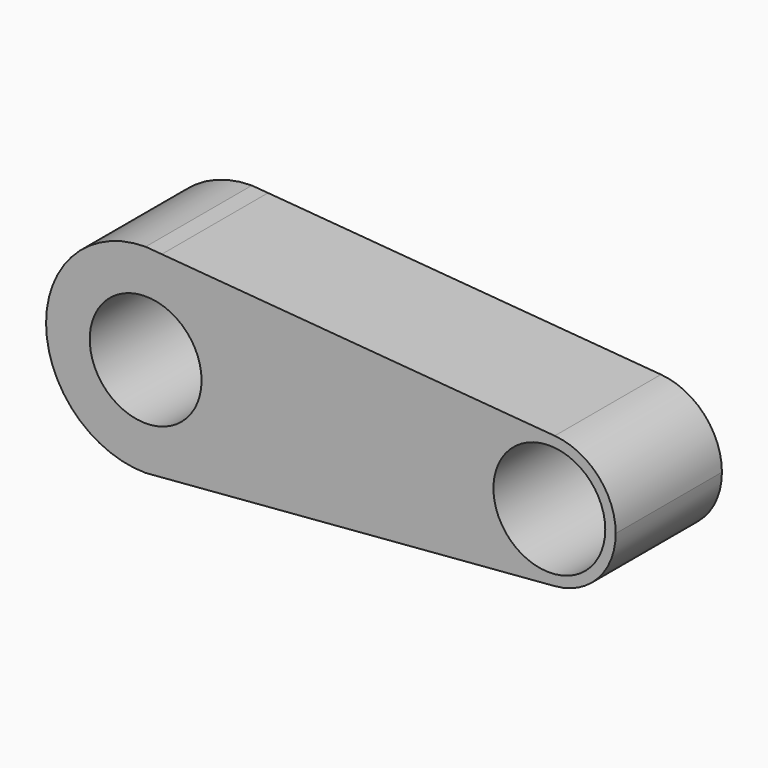
from build123d import *

# Parameters (mm, degrees)
F0_R     = 10.6986953421
F1_DEPTH = 25.4


with BuildPart() as f1:
    # F0 (on Front) → F1 (new body)
    with BuildSketch(Plane.XZ):
        with BuildLine():
            Line((3.0906604896, 18.7976146821), (0, 19.05))
            ThreePointArc((0, 19.05), (-19.05, 0), (0, -19.05))
            Line((0, -19.05), (3.0906604896, -18.7976146821))
            ThreePointArc((3.0906604896, -18.7976146821), (14.5220450063, -12.3293434065), (19.05, 0))
            ThreePointArc((19.05, 0), (14.5220450063, 12.3293434065), (3.0906604896, 18.7976146821))
        make_face()
        Circle(F0_R, mode=Mode.SUBTRACT)
        with BuildLine():
            Line((78.2768051379, 12.6578658873), (3.0906604896, 18.7976146821))
            ThreePointArc((3.0906604896, 18.7976146821), (14.5220450063, 12.3293434065), (19.05, 0))
            ThreePointArc((19.05, 0), (14.5220450063, -12.3293434065), (3.0906604896, -18.7976146821))
            Line((3.0906604896, -18.7976146821), (78.2768051379, -12.6578658873))
            ThreePointArc((78.2768051379, -12.6578658873), (64.5431556911, 0), (78.2768051379, 12.6578658873))
        make_face()
        with BuildLine():
            ThreePointArc((89.9431556911, 0), (86.5817141445, 8.6070509475), (78.2768051379, 12.6578658873))
            ThreePointArc((78.2768051379, 12.6578658873), (64.5431556911, 0), (78.2768051379, -12.6578658873))
            ThreePointArc((78.2768051379, -12.6578658873), (86.5817141445, -8.6070509475), (89.9431556911, 0))
        make_face()
        with Locations((77.2431556911, 0)):
            Circle(F0_R, mode=Mode.SUBTRACT)
    extrude(amount=F1_DEPTH)


solid = f1.part
